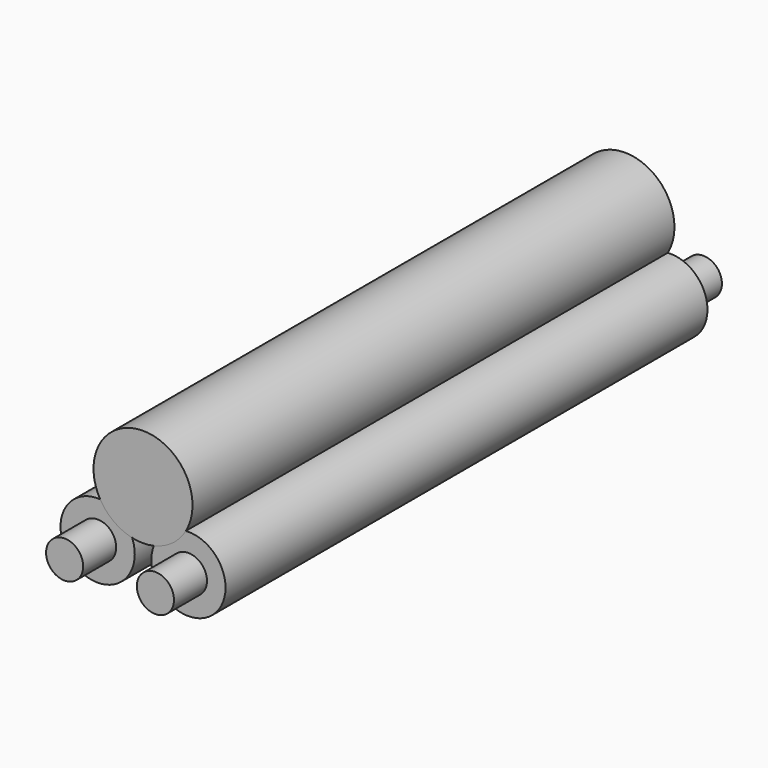
from build123d import *

# Parameters (mm, degrees)
F0_R          = 4.5
F1_DEPTH      = 36.5
F1_DEPTH_BACK = 36.5
F2_R          = 2.25
F3_DEPTH      = 41.5
F3_DEPTH_BACK = 41.5
F4_R          = 6
F5_DEPTH      = 36.5
F5_DEPTH_BACK = 36.5


with BuildPart() as f1:
    # F0 (on Front) → F1 (new body, two sides)
    with BuildSketch(Plane.XZ) as f1_sk:
        with Locations((-5.5, 0)):
            Circle(F0_R)
    extrude(amount=F1_DEPTH)
    extrude(f1_sk.sketch, amount=-F1_DEPTH_BACK)

    # F2 (on Front) → F3, piece 2 (join, two sides)
    with BuildSketch(Plane.XZ) as f3_2_sk:
        with Locations((-5.5, 0)):
            Circle(F2_R)
    extrude(amount=F3_DEPTH)
    extrude(f3_2_sk.sketch, amount=-F3_DEPTH_BACK)


with BuildPart() as f1b:
    # F0 (on Front) → F1, piece 2 (new body, two sides)
    with BuildSketch(Plane.XZ) as f1_2_sk:
        with Locations((5.5, 0)):
            Circle(F0_R)
    extrude(amount=F1_DEPTH)
    extrude(f1_2_sk.sketch, amount=-F1_DEPTH_BACK)

    # F2 (on Front) → F3 (join, two sides)
    with BuildSketch(Plane.XZ) as f3_sk:
        with Locations((5.5, 0)):
            Circle(F2_R)
    extrude(amount=F3_DEPTH)
    extrude(f3_sk.sketch, amount=-F3_DEPTH_BACK)


with BuildPart() as f5:
    # F4 (on Front) → F5 (new body, two sides)
    with BuildSketch(Plane.XZ) as f5_sk:
        with Locations((0, 7.5)):
            Circle(F4_R)
    extrude(amount=F5_DEPTH)
    extrude(f5_sk.sketch, amount=-F5_DEPTH_BACK)


solid = Compound([f1.part, f1b.part, f5.part])
